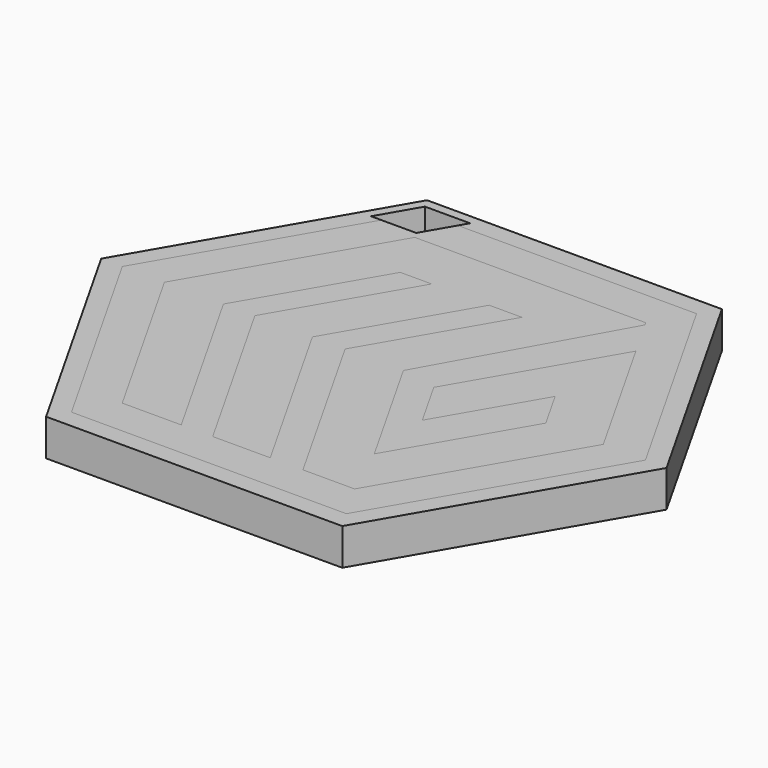
from build123d import *

# Parameters (mm, degrees)
F1_DEPTH  = 5
F3_DEPTH  = 5
F6_DEPTH  = 5
F8_DEPTH  = 25
F10_DEPTH = 25


# Not quite as in the source:
# - a feature names something its author has since deleted; it is built from what else it names


with BuildPart() as f1:
    # F0 (on Top) → F1 (new body)
    with BuildSketch(Plane.XY):
        Polygon((9.7598956231, -24.5410669595), (16.7959537357, -24.5410669595), (31.0372654349, 0), (20.3218720853, 18.9331807196), (8.7514274241, -1.0053658961), (12.5294908801, -7.6808798833), (20.1335282104, 5.4226314524), (23.2025122265, 0), (13.3824004213, -16.922319127), (3.8050711538, 0), (17.3130770462, 24.2494634137), (17.0587887483, 24.6987690194), (-14.4067760557, 24.6987690194), (-28.7396030991, 0), (-14.8503792237, -24.5410669595), (-6.8139773794, -24.5410669595), (-20.7032012548, 0), (-10.5808662515, 17.4431194507), (-6.2982602976, 17.4431194507), (-16.4205953009, 0), (-2.5313714255, -24.5410669595), (5.3053838201, -24.5410669595), (-8.5838400553, 0), (1.538494948, 17.4431194507), (5.9930067509, 17.4431194507), (-4.1293282523, 0), align=None)
    extrude(amount=F1_DEPTH)


with BuildPart() as f3:
    # F2 (on face) → F3 (new body)
    with BuildSketch(Plane.XY.offset(5)):
        Polygon((19.9742314443, 29.6987690194), (-17.2861539376, 29.6987690194), (-34.5024495524, 0.0311181456), (-17.7658219197, -29.5410669595), (19.6753316176, -29.5410669595), (36.8001118881, -0.0311181456), align=None)
    extrude(amount=-F3_DEPTH)

    # F4: cut F1
    add(f1.part, mode=Mode.SUBTRACT)

    # F7 (on face) → F8 (cut)
    with BuildSketch(Plane.XY.offset(5)):
        Polygon((-14.9207130098, 25.5912134556), (-12.5370766665, 29.6987690194), (-17.2861539376, 29.6987690194), (-19.6697902808, 25.5912134556), align=None)
    extrude(amount=-F8_DEPTH, mode=Mode.SUBTRACT)


with BuildPart() as f6:
    # F5 (on face) → F6 (new body, through all)
    with BuildSketch(Plane.XY.offset(5)):
        Polygon((21.4319527923, 32.1987690194), (-18.7258428786, 32.1987690194), (-37.383872779, 0.0466772184), (-19.2235432677, -32.0410669595), (21.1150205586, -32.0410669595), (39.6815351148, -0.0466772184), align=None)
        Polygon((-34.5024495524, 0.0311181456), (-17.2861539376, 29.6987690194), (19.9742314443, 29.6987690194), (36.8001118881, -0.0311181456), (19.6753316176, -29.5410669595), (-17.7658219197, -29.5410669595), align=None, mode=Mode.SUBTRACT)
    extrude(amount=-F6_DEPTH)

    # F9 (on face) → F10 (cut)
    with BuildSketch(Plane.XY.offset(5)):
        Polygon((-21.071260795, 25.5912134556), (-19.6697902808, 25.5912134556), (-14.9207130098, 25.5912134556), (-12.5370766665, 29.6987690194), (-11.8336566418, 30.9109240717), (-17.984204427, 30.9109240717), align=None)
    extrude(amount=-F10_DEPTH, mode=Mode.SUBTRACT)


solid = Compound([f1.part, f3.part, f6.part])
